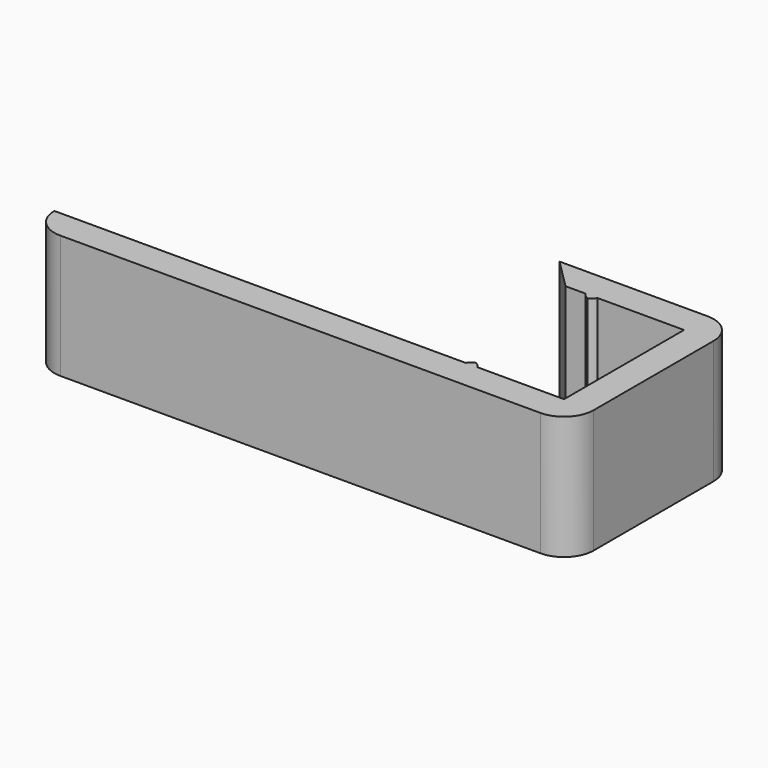
from build123d import *

# Parameters (mm, degrees)
F0_W         = 2
F0_H         = 1
F1_DEPTH     = 20.85
F2_SIZE      = 4.99999
F3_TEXT_SIZE = 16.6666666667
F4_DEPTH     = 1
F5_T1_DEPTH  = 29.5102540378


# Not quite as in the source:
# - a fillet or chamfer that OpenCascade refuses, or shapes differently, is made with other operations: its cross-section is extruded or revolved along the edge and cut away or added
# - a fillet or chamfer is up to 0.001 mm smaller than in the source, because OpenCascade refuses the exact size
# - Text() gives the source's letters only with a copy of the font that has no kerning and outlines rounded to 1/6400 em; it was checked with that copy


with BuildPart() as f1:
    # F0 (on Top) → F1 (new body)
    with BuildSketch(Plane.XY):
        with BuildLine():
            Line((-16.6, -12.65), (-86, -12.65))
            ThreePointArc((-86, -12.65), (-84.5355339059, -16.1855339059), (-81, -17.65))
            Line((-81, -17.65), (0, -17.65))
            ThreePointArc((0, -17.65), (3.5355339059, -16.1855339059), (5, -12.65))
            Line((5, -12.65), (5, 12.65))
            ThreePointArc((5, 12.65), (3.5355339059, 16.1855339059), (0, 17.65))
            Line((0, 17.65), (-25, 17.65))
            Line((-25, 17.65), (-25, 12.65))
            Line((-25, 12.65), (-16.6, 12.65))
            Line((-16.6, 12.65), (-14.6, 12.65))
            Line((-14.6, 12.65), (0, 12.65))
            Line((0, 12.65), (0, -12.65))
            Line((0, -12.65), (-14.6, -12.65))
            Line((-14.6, -12.65), (-16.6, -12.65))
        make_face()
        with Locations((-15.6, -12.15)):
            Rectangle(F0_W, F0_H)
        with Locations((-15.6, 12.15)):
            Rectangle(F0_W, F0_H)
    extrude(amount=F1_DEPTH)

    # F2 (size 5 in the source; OpenCascade refuses exactly that, so slightly less here)
    f2_edges = [f1.edges().sort_by_distance(p)[0] for p in [
        (-25, 12.65, 10.425),
    ]]
    chamfer(f2_edges, length=F2_SIZE)

    # F3 (on face) → F4 (cut)
    with BuildSketch(Plane(origin=(0, -12.65, 0), x_dir=(-1, 0, 0), z_dir=(0, 1, 0))):
        with Locations(Location((46, 16.425), (0, 0, 180))):
            Text('R', F3_TEXT_SIZE, font='Open Sans', font_style=FontStyle.BOLD, text_align=(TextAlign.LEFT, TextAlign.BOTTOM))
        Polygon((41.9791666667, 11.8598958333), (41.9791666667, 16.425), (37.796875, 16.425), (40.6380208333, 11.8598958333), align=None)
        with BuildLine():
            Line((41.9791666667, 6.5942708333), (41.9791666667, 9.8078125))
            Line((41.9791666667, 9.8078125), (41.1666666667, 9.8078125))
            add(Edge.make_bspline(
                [(41.1666666667, 9.8078125), (39.96875, 9.8078125), (39.3997395833, 9.409375)],
                knots=[0, 0, 0, 1, 1, 1], degree=2))
            add(Edge.make_bspline(
                [(39.3997395833, 9.409375), (38.8307291667, 9.0109375), (38.8307291667, 8.1567708333)],
                knots=[0, 0, 0, 1, 1, 1], degree=2))
            add(Edge.make_bspline(
                [(38.8307291667, 8.1567708333), (38.8307291667, 7.3104166667), (39.4127604167, 6.95234375)],
                knots=[0, 0, 0, 1, 1, 1], degree=2))
            add(Edge.make_bspline(
                [(39.4127604167, 6.95234375), (39.9947916667, 6.5942708333), (41.2135416667, 6.5942708333)],
                knots=[0, 0, 0, 1, 1, 1], degree=2))
            Line((41.2135416667, 6.5942708333), (41.9791666667, 6.5942708333))
        make_face()
    extrude(amount=-F4_DEPTH, mode=Mode.SUBTRACT)

    # F5: fillet of radius 2 on 4 edges, made by hand

    # F5_s2 → F5_t1 (cut)
    with BuildSketch(Plane.XY.offset(-4.3301270189)):
        with BuildLine():
            ThreePointArc((-16.6, 12.65), (-15.8679491924, 11.9179491924), (-14.8679491924, 11.65))
            Line((-14.8679491924, 11.65), (-16.6, 11.65))
            Line((-16.6, 11.65), (-16.6, 12.65))
        make_face()
        with BuildLine():
            ThreePointArc((-16.3320508076, 11.65), (-15.3320508076, 11.9179491924), (-14.6, 12.65))
            Line((-14.6, 12.65), (-14.6, 11.65))
            Line((-14.6, 11.65), (-16.3320508076, 11.65))
        make_face()
        with BuildLine():
            ThreePointArc((-16.6, -12.65), (-15.8679491924, -11.9179491924), (-14.8679491924, -11.65))
            Line((-14.8679491924, -11.65), (-16.6, -11.65))
            Line((-16.6, -11.65), (-16.6, -12.65))
        make_face()
        with BuildLine():
            ThreePointArc((-14.6, -12.65), (-15.3320508076, -11.9179491924), (-16.3320508076, -11.65))
            Line((-16.3320508076, -11.65), (-14.6, -11.65))
            Line((-14.6, -11.65), (-14.6, -12.65))
        make_face()
    extrude(amount=F5_T1_DEPTH, mode=Mode.SUBTRACT)


solid = f1.part
